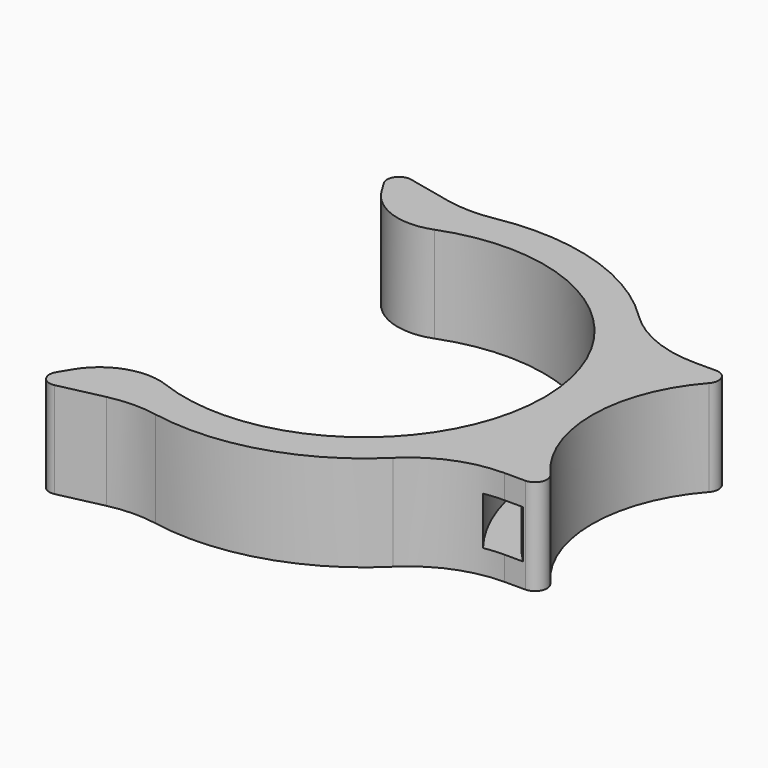
from build123d import *

# Parameters (mm, degrees)
F1_DEPTH = 8
F2_R     = 5
F3_R     = 1
F4_R     = 10
F7_DEPTH = 4
F8_R     = 1


# Not quite as in the source:
# - a feature names something its author has since deleted; it is built from what else it names


with BuildPart() as f1:
    # F0 (on Top) → F1 (new body)
    with BuildSketch(Plane.XY):
        with BuildLine():
            ThreePointArc((-2.9227996939, -0.1596333839), (-11.2678550126, -13.4433261015), (-26.890906557, -12.0232201439))
            Line((-26.890906557, -12.0232201439), (-31.1837848276, -19.0931353718))
            Line((-31.1837848276, -19.0931353718), (-22.9890488593, -17.2720731705))
            ThreePointArc((-22.9890488593, -17.2720731705), (-11.7519193442, -16.909486057), (-2.9219502426, -9.9498743711))
            Line((-2.9219502426, -9.9498743711), (6.0116767822, -9.9498743711))
            ThreePointArc((6.0116767822, -9.9498743711), (1.0780497574, 0), (6.0116767822, 9.9498743711))
            Line((6.0116767822, 9.9498743711), (-2.9219502426, 9.9498743711))
            ThreePointArc((-2.9219502426, 9.9498743711), (-11.7519193442, 16.909486057), (-22.9890488593, 17.2720731705))
            Line((-22.9890488593, 17.2720731705), (-31.1837848276, 19.0931353718))
            Line((-31.1837848276, 19.0931353718), (-26.890906557, 12.0232201439))
            ThreePointArc((-26.890906557, 12.0232201439), (-11.3609432233, 13.4890024425), (-2.9264400932, 0.3669814152))
            Line((-2.9264400932, 0.3669814152), (-2.9219502426, 0.3647975664))
            Line((-2.9219502426, 0.3647975664), (-2.9219502426, -3.27e-08))
            Line((-2.9219502426, -3.27e-08), (-2.9219502426, -0.1592372783))
            Line((-2.9219502426, -0.1592372783), (-2.9227996939, -0.1596333839))
        make_face()
        with BuildLine():
            ThreePointArc((-2.9219502426, -3.27e-08), (-2.922162607, -0.0798178383), (-2.9227996939, -0.1596333839))
            Line((-2.9227996939, -0.1596333839), (-2.9219502426, -0.1592372783))
            Line((-2.9219502426, -0.1592372783), (-2.9219502426, -3.27e-08))
        make_face()
        with BuildLine():
            ThreePointArc((-2.9264400932, 0.3669814152), (-2.923072747, 0.1835044236), (-2.9219502426, -3.27e-08))
            Line((-2.9219502426, -3.27e-08), (-2.9219502426, 0.3647975664))
            Line((-2.9219502426, 0.3647975664), (-2.9264400932, 0.3669814152))
        make_face()
    extrude(amount=F1_DEPTH)

    # F2
    f2_edges = [f1.edges().sort_by_distance(p)[0] for p in [
        (-26.890907, 12.02322, 4),
        (-26.890907, -12.02322, 4),
    ]]
    fillet(f2_edges, radius=F2_R)

    # F3
    f3_edges = [f1.edges().sort_by_distance(p)[0] for p in [
        (-31.183785, -19.093135, 4),
        (-31.183785, 19.093135, 4),
    ]]
    fillet(f3_edges, radius=F3_R)

    # F4
    f4_edges = [f1.edges().sort_by_distance(p)[0] for p in [
        (-2.92195, 9.949874, 4),
        (-2.92195, -9.949874, 4),
        (-22.989049, 17.272073, 4),
        (-22.989049, -17.272073, 4),
    ]]
    fillet(f4_edges, radius=F4_R)

    # F6 (on offset) → F7 (cut)
    with BuildSketch(Plane.XY.offset(6)):
        with BuildLine():
            ThreePointArc((11.3967054025, -13.8123607251), (-0.7746921386, -2.0181552322), (7.4959259895, 12.7751904709))
            Line((7.4959259895, 12.7751904709), (2.6926121721, 12.7751904709))
            ThreePointArc((2.6926121721, 12.7751904709), (-3.3979094134, -0.8877509035), (4.1336827916, -13.8123607251))
            Line((4.1336827916, -13.8123607251), (11.3967054025, -13.8123607251))
        make_face()
    extrude(amount=-F7_DEPTH, mode=Mode.SUBTRACT)

    # F8
    f8_edges = [f1.edges().sort_by_distance(p)[0] for p in [
        (6.011677, 9.949874, 4),
        (6.011677, -9.949874, 4),
    ]]
    fillet(f8_edges, radius=F8_R)


solid = f1.part
